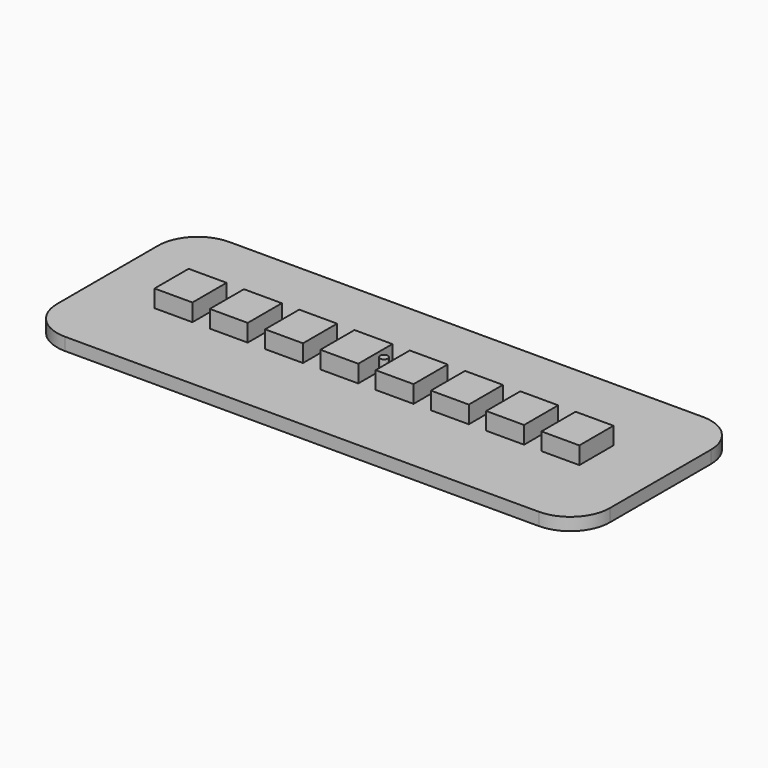
from build123d import *

# Parameters (mm, degrees)
F0_W     = 35
F0_H     = 13
F1_DEPTH = 0.8
F2_W     = 2.4
F2_H     = 2.7
F3_DEPTH = 1.1
F4_R     = 2.5
F5_R     = 0.25
F6_DEPTH = 1.1


# Not quite as in the source:
# - a feature names something its author has since deleted; it is built from what else it names


with BuildPart() as f1:
    # F0 (on Top) → F1 (new body)
    with BuildSketch(Plane.XY):
        Rectangle(F0_W, F0_H)
    extrude(amount=F1_DEPTH)

    # F2 (on face) → F3 (join)
    with BuildSketch(Plane.XY.offset(0.8)):
        with Locations((-12.25, 0)):
            Rectangle(F2_W, F2_H)
        with Locations((-8.75, 0)):
            Rectangle(F2_W, F2_H)
        with Locations((-5.25, 0)):
            Rectangle(F2_W, F2_H)
        with Locations((-1.75, 0)):
            Rectangle(F2_W, F2_H)
        with Locations((1.75, 0)):
            Rectangle(F2_W, F2_H)
        with Locations((5.25, 0)):
            Rectangle(F2_W, F2_H)
        with Locations((8.75, 0)):
            Rectangle(F2_W, F2_H)
        with Locations((12.25, 0)):
            Rectangle(F2_W, F2_H)
    extrude(amount=F3_DEPTH)

    # F4
    f4_edges = [f1.edges().sort_by_distance(p)[0] for p in [
        (-17.5, 6.5, 0.4),
        (-17.5, -6.5, 0.4),
        (17.5, -6.5, 0.4),
        (17.5, 6.5, 0.4),
    ]]
    fillet(f4_edges, radius=F4_R)

    # F5 (on face) → F6 (join)
    with BuildSketch(Plane.XY.offset(0.8)):
        Circle(F5_R)
    extrude(amount=F6_DEPTH)


solid = f1.part
